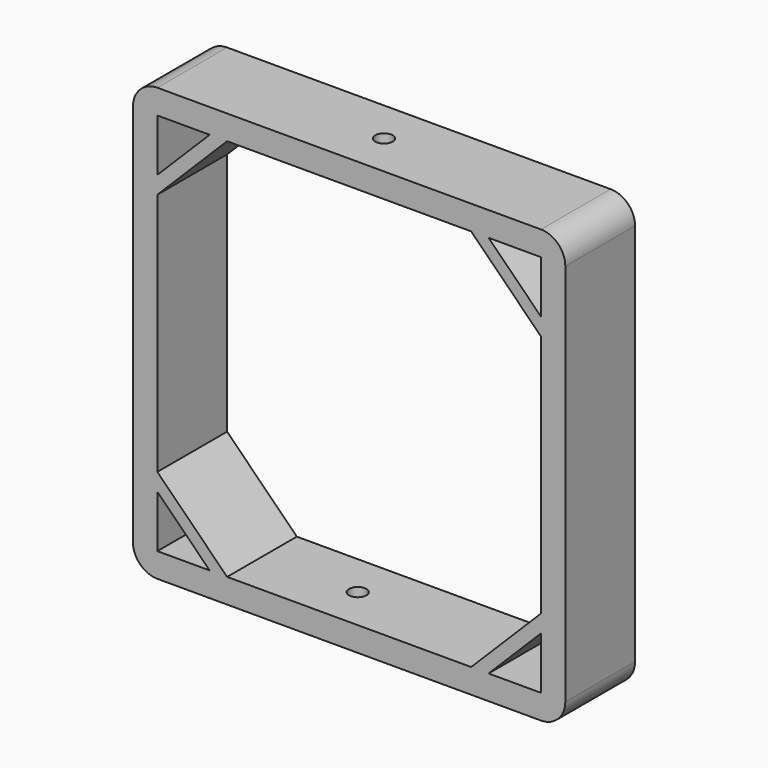
from build123d import *

# Parameters (mm, degrees)
F1_DEPTH = 25
F3_R     = 2.5
F4_DEPTH = 25
F2_R     = 2.5
F5_DEPTH = 25


# Not quite as in the source:
# - ends of sketch curves that miss each other by under 0.0002 mm in the source are joined


with BuildPart() as f1:
    # F0 (on Front) → F1 (new body)
    with BuildSketch(Plane.XZ):
        with BuildLine():
            Line((40, 55), (55, 55))
            Line((55, 55), (55, 62.0000141774))
            Line((55, 62.0000141774), (-55, 62.0000141774))
            ThreePointArc((-55, 62.0000141774), (-59.9497599972, 59.9497599972), (-62.0000177185, 55))
            Line((-62.0000177185, 55), (-62.0000141774, -55))
            ThreePointArc((-62.0000141774, -55), (-59.9497574932, -59.9497574932), (-55, -62.0000141774))
            Line((-55, -62.0000141774), (-55, -55))
            Line((-55, -55), (-55, -40))
            Line((-55, -40), (-55, -35))
            Line((-55, -35), (-55, 35))
            Line((-55, 35), (-55, 40))
            Line((-55, 40), (-55, 55))
            Line((-55, 55), (-40, 55))
            Line((-40, 55), (-35, 55))
            Line((-35, 55), (35, 55))
            Line((35, 55), (40, 55))
        make_face()
        with BuildLine():
            Line((55, 62.0000141774), (55, 55))
            Line((55, 55), (55, 40))
            Line((55, 40), (55, 35))
            Line((55, 35), (55, -35))
            Line((55, -35), (55, -40))
            Line((55, -40), (55, -55))
            Line((55, -55), (40, -55))
            Line((40, -55), (35, -55))
            Line((35, -55), (-35, -55))
            Line((-35, -55), (-40, -55))
            Line((-40, -55), (-55, -55))
            Line((-55, -55), (-55, -62.0000141774))
            Line((-55, -62.0000141774), (55, -62.0000141774))
            ThreePointArc((55, -62.0000141774), (59.9497599972, -59.9497599972), (62.0000177185, -55))
            Line((62.0000177185, -55), (62.0000141774, 55))
            ThreePointArc((62.0000141774, 55), (59.9497574932, 59.9497574932), (55, 62.0000141774))
        make_face()
        Polygon((-55, 35), (-35, 55), (-40, 55), (-55, 40), align=None)
        Polygon((55, 40), (40, 55), (35, 55), (55, 35), align=None)
        Polygon((55, -40), (55, -35), (35, -55), (40, -55), align=None)
        Polygon((-35, -55), (-55, -35), (-55, -40), (-40, -55), align=None)
    extrude(amount=F1_DEPTH)

    # F3 (on face) → F4 (cut)
    with BuildSketch(Plane(origin=(0, 0, -62.0000141774), x_dir=(1, 0, 0), z_dir=(0, 0, -1))):
        with Locations((-7.5450468063, 12.5)):
            Circle(F3_R)
    extrude(amount=-F4_DEPTH, mode=Mode.SUBTRACT)

    # F2 (on face) → F5 (cut)
    with BuildSketch(Plane.XY.offset(62.0000141774)):
        with Locations((0, -12.5)):
            Circle(F2_R)
    extrude(amount=-F5_DEPTH, mode=Mode.SUBTRACT)


solid = f1.part
